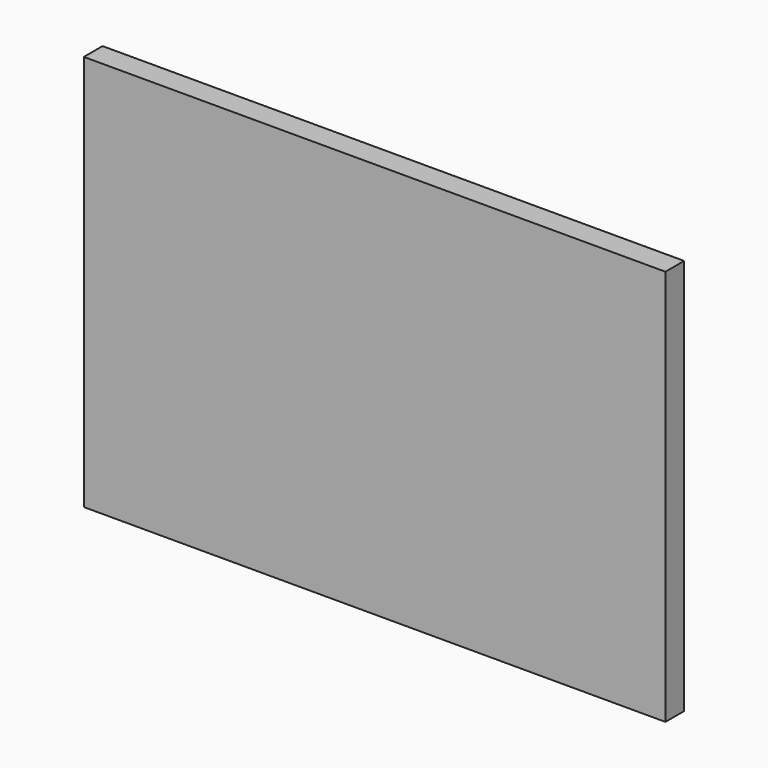
from build123d import *

# Parameters (mm, degrees)
F1_W           = 99.3780978024
F1_H           = 67.7224099636
F2_DEPTH       = 6
F0_W           = 8
F0_H           = 56
F3_DEPTH       = 3
F4_TEXT_SIZE   = 9.8900798346
F4_TEXT_SIZE_2 = 9.8611111111
F4_TEXT_SIZE_3 = 10.1897787924
F4_TEXT_SIZE_4 = 10.9390265101
F5_DEPTH       = 0.5
F6_W           = 3
F6_H           = 3
F6_W_2         = 93.3780978024
F6_H_2         = 61.7224099636
F7_DEPTH       = 2


# Not quite as in the source:
# - Text() gives the source's letters only with a copy of the font that has no kerning and outlines rounded to 1/6400 em; it was checked with that copy


with BuildPart() as f2:
    # F1 (on Front) → F2 (new body)
    with BuildSketch(Plane.XZ):
        with Locations((-2.98393704, 4.2813010514)):
            Rectangle(F1_W, F1_H)
    extrude(amount=F2_DEPTH)

    # F0 (on Front) → F3 (cut)
    with BuildSketch(Plane.XZ):
        with Locations((-40.7372321934, 4.2707970198)):
            Rectangle(F0_W, F0_H)
        with Locations((-26.4214153439, 4.4369018376)):
            Rectangle(F0_W, F0_H)
        with Locations((-13.2214191407, 4.4369018376)):
            Rectangle(F0_W, F0_H)
        with Locations((-1.2999998443, 4.4569811523)):
            Rectangle(F0_W, F0_H)
        with Locations((9.600000266, 4.4569811523)):
            Rectangle(F0_W, F0_H)
        with Locations((21.3067618161, 4.1268533766)):
            Rectangle(F0_W, F0_H)
        with Locations((34.2729867399, 4.1853348464)):
            Rectangle(F0_W, F0_H)
    extrude(amount=F3_DEPTH, mode=Mode.SUBTRACT)

    # F4 (on face) → F5 (cut)
    with BuildSketch(Plane(origin=(0, -3, 0), x_dir=(-1, 0, 0), z_dir=(0, 1, 0))):
        with Locations((-36.5318208933, 6.2568751164)):
            Text('1', F4_TEXT_SIZE, font='Open Sans', text_align=(TextAlign.LEFT, TextAlign.BOTTOM))
        with Locations((-24.0440241426, 6.4935181752)):
            Text('2', F4_TEXT_SIZE_2, font='Open Sans', text_align=(TextAlign.LEFT, TextAlign.BOTTOM))
        with Locations((-12.1482796967, 6.5805502236)):
            Text('3', F4_TEXT_SIZE_3, font='Open Sans', text_align=(TextAlign.LEFT, TextAlign.BOTTOM))
        with Locations((-1.790668699, 6.7963339388)):
            Text('4', F4_TEXT_SIZE_3, font='Open Sans', text_align=(TextAlign.LEFT, TextAlign.BOTTOM))
        with Locations((9.9695343524, 6.6884420812)):
            Text('5', F4_TEXT_SIZE_4, font='Open Sans', text_align=(TextAlign.LEFT, TextAlign.BOTTOM))
        with Locations((23.748242465, 7.1408674583)):
            Text('6', F4_TEXT_SIZE_2, font='Open Sans', text_align=(TextAlign.LEFT, TextAlign.BOTTOM))
        with Locations((38.0700540107, 7.5724339575)):
            Text('7', F4_TEXT_SIZE_2, font='Open Sans', text_align=(TextAlign.LEFT, TextAlign.BOTTOM))
    extrude(amount=-F5_DEPTH, mode=Mode.SUBTRACT)

    # F6 (on face) → F7 (cut)
    with BuildSketch(Plane(origin=(0, 0, 0), x_dir=(-1, 0, 0), z_dir=(0, 1, 0))):
        with Locations((-45.2051118612, 36.6425060332)):
            Rectangle(F6_W, F6_H)
        with Locations((2.98393704, 36.6425060332)):
            Rectangle(F6_W_2, F6_H)
        with Locations((-45.2051118612, 4.2813010514)):
            Rectangle(F6_W, F6_H_2)
        with Locations((51.1729859412, 36.6425060332)):
            Rectangle(F6_W, F6_H)
        with Locations((-45.2051118612, -28.0799039304)):
            Rectangle(F6_W, F6_H)
        with Locations((51.1729859412, 4.2813010514)):
            Rectangle(F6_W, F6_H_2)
        with Locations((2.98393704, -28.0799039304)):
            Rectangle(F6_W_2, F6_H)
        with Locations((51.1729859412, -28.0799039304)):
            Rectangle(F6_W, F6_H)
    extrude(amount=-F7_DEPTH, mode=Mode.SUBTRACT)


with BuildPart() as f8_1:
    # F8: copy of F2
    add(f2.part)


solid = Compound([f2.part, f8_1.part])
